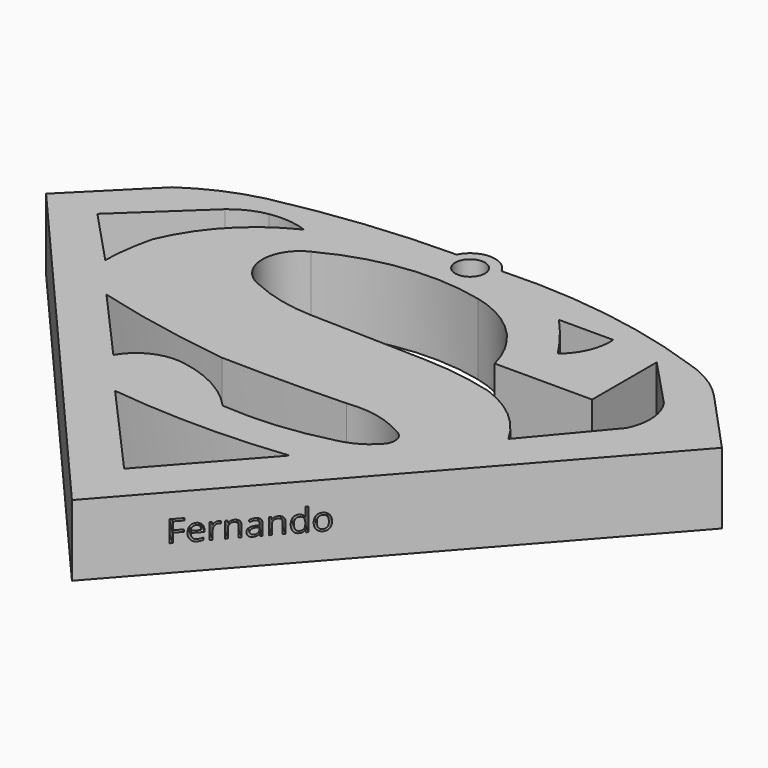
from build123d import *

# Parameters (mm, degrees)
F0_R         = 1.044319326
F1_DEPTH     = 5
F2_TEXT_SIZE = 2.0902966046
F3_DEPTH     = 2


# Not quite as in the source:
# - Text() gives the source's letters only with a copy of the font that has no kerning and outlines rounded to 1/6400 em; it was checked with that copy


with BuildPart() as f1:
    # F0 (on Top) → F1 (new body)
    with BuildSketch(Plane.XY):
        with BuildLine():
            Line((1.1784326052, 28.3566471189), (25.0625759363, 0.7754490362))
            Line((25.0625759363, 0.7754490362), (49.0640886128, 27.945863083))
            Line((49.0640886128, 27.945863083), (44.8975674808, 32.4644856155))
            ThreePointArc((44.8975674808, 32.4644856155), (43.3394495955, 33.7523043815), (41.4939299226, 34.5770865679))
            ThreePointArc((41.4939299226, 34.5770865679), (34.0911792639, 36.4139339047), (26.4735481716, 36.7965851754))
            ThreePointArc((26.4735481716, 36.7965851754), (24.8939363417, 37.7688306275), (23.3177434192, 36.7910522155))
            ThreePointArc((23.3177434192, 36.7910522155), (17.1136377912, 36.4435140258), (10.9785608947, 35.4573391378))
            ThreePointArc((10.9785608947, 35.4573391378), (8.4424620528, 34.5976753466), (6.1078383587, 33.2860536873))
            Line((6.1078383587, 33.2860536873), (1.1784326052, 28.3566471189))
        make_face()
        with BuildLine():
            Line((24.9674525112, 5.4851286113), (18.7910236418, 12.4097699299))
            ThreePointArc((18.7910236418, 12.4097699299), (24.9372698645, 12.0429787611), (31.0851968825, 12.3804276809))
            Line((31.0851968825, 12.3804276809), (24.9674525112, 5.4851286113))
        make_face(mode=Mode.SUBTRACT)
        with BuildLine():
            Line((16.0498730838, 15.6823787838), (11.269482784, 21.0559554398))
            ThreePointArc((11.269482784, 21.0559554398), (16.0664109822, 19.9354363901), (20.9305826575, 19.1570296884))
            ThreePointArc((20.9305826575, 19.1570296884), (25.2946564349, 19.1122489615), (29.6582821757, 19.1891621798))
            ThreePointArc((29.6582821757, 19.1891621798), (31.8255432811, 19.1065629757), (33.8454842567, 18.3168277144))
            ThreePointArc((33.8454842567, 18.3168277144), (34.4848062837, 17.6140493014), (34.2467576265, 16.6942868382))
            ThreePointArc((34.2467576265, 16.6942868382), (33.2173387817, 15.8587065792), (31.9786928594, 15.3857860714))
            ThreePointArc((31.9786928594, 15.3857860714), (28.2734124243, 14.7354412232), (24.5115123689, 14.7228119895))
            ThreePointArc((24.5115123689, 14.7228119895), (22.3242387564, 16.4367893027), (19.6962300688, 17.3398144543))
            ThreePointArc((19.6962300688, 17.3398144543), (17.6106906268, 17.088290472), (16.0498730838, 15.6823787838))
        make_face(mode=Mode.SUBTRACT)
        with BuildLine():
            Line((8.6506521329, 24.2228601128), (4.8756320029, 28.2446127385))
            Line((4.8756320029, 28.2446127385), (10.0076850504, 33.0559127033))
            ThreePointArc((10.0076850504, 33.0559127033), (11.0605863233, 33.733968384), (12.2529584914, 34.1168642044))
            ThreePointArc((12.2529584914, 34.1168642044), (13.6015976662, 34.1693190355), (14.9176772684, 33.8701307774))
            ThreePointArc((14.9176772684, 33.8701307774), (11.4716424449, 31.367286809), (9.144118987, 27.8004929423))
            ThreePointArc((9.144118987, 27.8004929423), (8.7971146113, 26.0255070104), (8.6506521329, 24.2228601128))
        make_face(mode=Mode.SUBTRACT)
        with Locations((24.8970296234, 36.0045321286)):
            Circle(F0_R, mode=Mode.SUBTRACT)
        with BuildLine():
            Line((39.9117618799, 27.9732067138), (39.9117618799, 33.648069948))
            Line((39.9117618799, 33.648069948), (43.2426594198, 30.119786039))
            ThreePointArc((43.2426594198, 30.119786039), (43.8703480409, 28.3406037221), (43.4893928468, 26.4928061515))
            Line((43.4893928468, 26.4928061515), (39.2455793917, 21.4347727597))
            ThreePointArc((39.2455793917, 21.4347727597), (37.3672996149, 23.7250107349), (34.8043814301, 25.2097919583))
            ThreePointArc((34.8043814301, 25.2097919583), (32.3450752959, 25.7240008846), (29.8421127395, 25.9425779263))
            Line((29.8421127395, 25.9425779263), (21.5301290154, 26.1720530689))
            ThreePointArc((21.5301290154, 26.1720530689), (19.2691286683, 26.4654294427), (17.1136036515, 27.2083319724))
            ThreePointArc((17.1136036515, 27.2083319724), (15.3452989273, 29.5551560667), (16.8668702245, 32.0689789951))
            ThreePointArc((16.8668702245, 32.0689789951), (22.0595683818, 33.7223780176), (27.5010764599, 33.4260128438))
            ThreePointArc((27.5010764599, 33.4260128438), (31.04450693, 31.4811855904), (33.0525748432, 27.9732067138))
            Line((33.0525748432, 27.9732067138), (39.9117618799, 27.9732067138))
        make_face(mode=Mode.SUBTRACT)
        with BuildLine():
            ThreePointArc((35.0264422596, 31.0573726892), (33.8567036418, 32.6983588403), (32.5591079891, 34.2402309179))
            Line((32.5591079891, 34.2402309179), (36.383472383, 34.2402309179))
            ThreePointArc((36.383472383, 34.2402309179), (36.089937809, 32.4846631328), (35.0264422596, 31.0573726892))
        make_face(mode=Mode.SUBTRACT)
    extrude(amount=F1_DEPTH)

    # F2 (on face) → F3 (cut)
    with BuildSketch(Plane(origin=(13.6926357856, -12.0956556207, 0), x_dir=(0.6620498586, 0.7494597953, 0), z_dir=(0.7494597953, -0.6620498586, 0))):
        with Locations((22.4242992699, 1.8346612342)):
            Text('Fernando', F2_TEXT_SIZE, font='Open Sans', text_align=(TextAlign.LEFT, TextAlign.BOTTOM))
    extrude(amount=-F3_DEPTH, mode=Mode.SUBTRACT)


solid = f1.part
